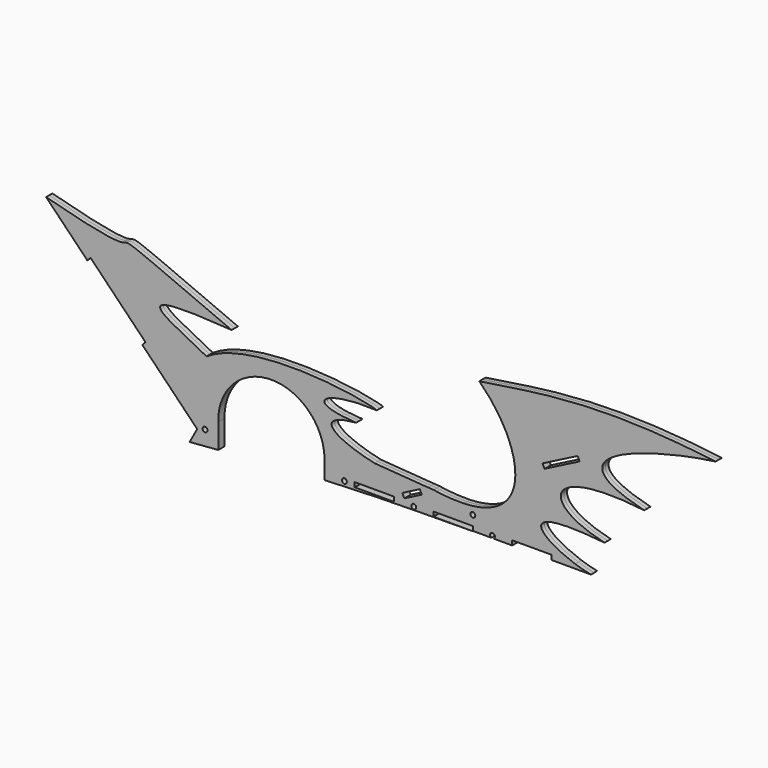
from build123d import *

# Parameters (mm, degrees)
F0_R     = 1.5875
F1_DEPTH = 2.54
F2_DEPTH = 2.54


# Not quite as in the source:
# - a feature names something its author has since deleted; it is built from what else it names


with BuildPart() as f1:
    # F0 (on Front) → F1 (new body)
    with BuildSketch(Plane.XZ):
        with BuildLine():
            Line((-117.7666419361, -55.4287118418), (-109.9768313618, -55.4287118418))
            Line((-109.9768313618, -55.4287118418), (-109.9768313618, -47.0136375922))
            ThreePointArc((-109.9768313618, -47.0136375922), (-106.8885192596, -31.8588641059), (-97.4549951083, -19.6027043016))
            add(Edge.make_bspline(
                [(-117.5484094073, -12.1659971935), (-110.6681944827, -14.9321483823), (-103.9782175093, -17.3987240026), (-97.4549951083, -19.6027043016)],
                knots=[85.5800903731, 85.5800903731, 85.5800903731, 85.5800903731, 105.0897215055, 105.0897215055, 105.0897215055, 105.0897215055], degree=3))
            add(Edge.make_bspline(
                [(-221.0534861924, 44.6501588425), (-181.5698408099, 17.8661525637), (-147.728857773, -0.032119976), (-117.5484094073, -12.1659971935)],
                knots=[0, 0, 0, 0, 85.5800903731, 85.5800903731, 85.5800903731, 85.5800903731], degree=3))
            Line((-221.0534861924, 44.6501588425), (-194.470886592, 17.3559213832))
            Line((-194.470886592, 17.3559213832), (-192.3419360702, 19.429364152))
            Line((-192.3419360702, 19.429364152), (-156.8984699364, -16.9629524605))
            Line((-156.8984699364, -16.9629524605), (-159.0274204582, -19.0363952293))
            Line((-159.0274204582, -19.0363952293), (-123.5839543244, -55.4287118418))
            Line((-123.5839543244, -55.4287118418), (-119.2412667127, -55.4287118418))
            ThreePointArc((-119.2412667127, -55.4287118418), (-119.3254386011, -52.6643963439), (-116.9164543244, -54.0228218418))
            ThreePointArc((-116.9164543244, -54.0228218418), (-117.1455288266, -54.8443061184), (-117.7666419361, -55.4287118418))
        make_face()
        with BuildLine():
            ThreePointArc((-97.4549951083, -19.6027043016), (-67.2988267393, -12.8616988757), (-43.9640451784, -33.1181451176))
            add(Edge.make_bspline(
                [(-43.9640451784, -33.1181451176), (-32.0425687929, -35.1610667408), (-20.543079457, -36.5394679062), (-9.2562094033, -37.5830486955)],
                knots=[162.0898574654, 162.0898574654, 162.0898574654, 162.0898574654, 202.5442303334, 202.5442303334, 202.5442303334, 202.5442303334], degree=3))
            add(Edge.make_bspline(
                [(-21.0130102932, -18.435029313), (-47.6523786783, -20.7854453474), (-38.7050335474, -30.7782148652), (-9.2562094033, -37.5830486955)],
                knots=[0, 0, 0, 0, 22.4692904525, 22.4692904525, 22.4692904525, 22.4692904525], degree=3))
            add(Edge.make_bspline(
                [(-7.7310134657, -7.0962994359), (-41.7368360795, -5.3299111314), (-56.8069815636, -16.3296777755), (-21.0130102932, -18.435029313)],
                knots=[0, 0, 0, 0, 17.4636260539, 17.4636260539, 17.4636260539, 17.4636260539], degree=3))
            add(Edge.make_bspline(
                [(-117.5484094073, -12.1659971935), (-86.6610095747, 8.189654137), (-15.093958471, -3.4407672938), (-7.7310134657, -7.0962994359)],
                knots=[0, 0, 0, 0, 109.9343544428, 109.9343544428, 109.9343544428, 109.9343544428], degree=3))
            add(Edge.make_bspline(
                [(-117.5484094073, -12.1659971935), (-110.6681944827, -14.9321483823), (-103.9782175093, -17.3987240026), (-97.4549951083, -19.6027043016)],
                knots=[85.5800903731, 85.5800903731, 85.5800903731, 85.5800903731, 105.0897215055, 105.0897215055, 105.0897215055, 105.0897215055], degree=3))
        make_face()
        with BuildLine():
            Line((-27.9141419361, -55.4287118418), (-21.9839543244, -55.4287118418))
            Line((-21.9839543244, -55.4287118418), (-21.9839543244, -52.4569118418))
            Line((-21.9839543244, -52.4569118418), (3.4160456756, -52.4569118418))
            Line((3.4160456756, -52.4569118418), (3.4160456756, -55.4287118418))
            Line((3.4160456756, -55.4287118418), (15.3787332873, -55.4287118418))
            ThreePointArc((15.3787332873, -55.4287118418), (15.2945613989, -52.6643963439), (17.7035456756, -54.0228218418))
            ThreePointArc((17.7035456756, -54.0228218418), (17.4744711734, -54.8443061184), (16.8533580639, -55.4287118418))
            Line((16.8533580639, -55.4287118418), (28.8160456756, -55.4287118418))
            Line((28.8160456756, -55.4287118418), (28.8160456756, -52.6365224585))
            Line((28.8160456756, -52.6365224585), (54.2160456756, -52.6365224585))
            Line((54.2160456756, -52.6365224585), (54.2160456756, -55.4287118418))
            Line((54.2160456756, -55.4287118418), (66.1787332873, -55.4287118418))
            ThreePointArc((66.1787332873, -55.4287118418), (66.0945613989, -52.6643963439), (68.5035456756, -54.0228218418))
            ThreePointArc((68.5035456756, -54.0228218418), (68.2744711734, -54.8443061184), (67.6533580639, -55.4287118418))
            Line((67.6533580639, -55.4287118418), (79.6160456756, -55.4287118418))
            Line((79.6160456756, -55.4287118418), (79.6160456756, -52.4715288512))
            Line((79.6160456756, -52.4715288512), (105.0160456756, -52.4715288512))
            Line((105.0160456756, -52.4715288512), (105.0160456756, -55.4287118418))
            Line((105.0160456756, -55.4287118418), (130.4160456756, -55.4287118418))
            add(Edge.make_bspline(
                [(130.4160456756, -55.4287118418), (127.0833152181, -54.7907548199), (123.567769086, -53.8343331493), (120.1337166001, -52.6704820922)],
                knots=[0, 0, 0, 0, 2.981631712, 2.981631712, 2.981631712, 2.981631712], degree=3))
            add(Edge.make_bspline(
                [(48.3758309171, -41.6905821706), (71.0941321723, -43.4592939375), (94.4273288023, -46.1963068791), (120.1337166001, -52.6704820922)],
                knots=[272.3833290429, 272.3833290429, 272.3833290429, 272.3833290429, 354.6125504281, 354.6125504281, 354.6125504281, 354.6125504281], degree=3))
            add(Edge.make_bspline(
                [(48.3758309171, -41.6905821706), (43.2278307913, -41.8740335792), (37.4162620901, -41.5445708983), (30.8966081292, -40.6238344152)],
                knots=[68.7701344649, 68.7701344649, 68.7701344649, 68.7701344649, 76.3944524282, 76.3944524282, 76.3944524282, 76.3944524282], degree=3))
            Line((30.8966081292, -40.6238344152), (21.3371492148, -45.5034172427))
            Line((21.3371492148, -45.5034172427), (10.0255792014, -51.277357304))
            Line((10.0255792014, -51.277357304), (8.674477227, -48.6304499209))
            Line((8.674477227, -48.6304499209), (19.9860472404, -42.8565098596))
            Line((19.9860472404, -42.8565098596), (25.3584616646, -40.1141850689))
            add(Edge.make_bspline(
                [(-9.2562094033, -37.5830486955), (2.4325313973, -38.6637863394), (13.8932426879, -39.3854364842), (25.3584616646, -40.1141850689)],
                knots=[202.5442303334, 202.5442303334, 202.5442303334, 202.5442303334, 244.4389873788, 244.4389873788, 244.4389873788, 244.4389873788], degree=3))
            add(Edge.make_bspline(
                [(-43.9640451784, -33.1181451176), (-32.0425687929, -35.1610667408), (-20.543079457, -36.5394679062), (-9.2562094033, -37.5830486955)],
                knots=[162.0898574654, 162.0898574654, 162.0898574654, 162.0898574654, 202.5442303334, 202.5442303334, 202.5442303334, 202.5442303334], degree=3))
            ThreePointArc((-43.9640451784, -33.1181451176), (-42.0894588544, -39.308762747), (-41.4107711408, -45.7412741932))
            ThreePointArc((-41.4107711408, -45.7412741932), (-41.4093090413, -45.924090419), (-41.4088216702, -46.1069118418))
            ThreePointArc((-41.4088216702, -46.1069118418), (-41.4093090413, -46.2897332645), (-41.4107711408, -46.4725494903))
            Line((-41.4107711408, -46.4725494903), (-41.4107711408, -55.4287118418))
            Line((-41.4107711408, -55.4287118418), (-29.3887667127, -55.4287118418))
            ThreePointArc((-29.3887667127, -55.4287118418), (-29.4729386011, -52.6643963439), (-27.0639543244, -54.0228218418))
            ThreePointArc((-27.0639543244, -54.0228218418), (-27.2930288266, -54.8443061184), (-27.9141419361, -55.4287118418))
        make_face()
        with Locations((54.2160456756, -46.2865224585)):
            Circle(F0_R, mode=Mode.SUBTRACT)
        with BuildLine():
            Line((-109.9768313618, -62.8472353007), (-109.9768313618, -55.4287118418))
            Line((-109.9768313618, -55.4287118418), (-117.7666419361, -55.4287118418))
            ThreePointArc((-117.7666419361, -55.4287118418), (-118.5039543244, -55.6103218418), (-119.2412667127, -55.4287118418))
            Line((-119.2412667127, -55.4287118418), (-123.5839543244, -55.4287118418))
            Line((-123.5839543244, -55.4287118418), (-128.4894852792, -64.325979178))
            add(Edge.make_bspline(
                [(-128.4894852792, -64.325979178), (-121.7990702135, -63.8053858531), (-115.6687309059, -63.3129022925), (-109.9768313618, -62.8472353007)],
                knots=[0, 0, 0, 0, 19.3690037374, 19.3690037374, 19.3690037374, 19.3690037374], degree=3))
        make_face()
        with BuildLine():
            add(Edge.make_bspline(
                [(58.3871234256, 30.9589318931), (71.6334399841, 18.2907250781), (80.3919593775, 2.3020275424), (81.5074353868, -11.4531938545)],
                knots=[0, 0, 0, 0, 31.5527935417, 31.5527935417, 31.5527935417, 31.5527935417], degree=3))
            Line((81.5074353868, -11.4531938545), (99.1670373344, -2.4389294304))
            Line((99.1670373344, -2.4389294304), (121.7901773612, 9.1089506922))
            Line((121.7901773612, 9.1089506922), (123.1412793355, 6.4620433091))
            Line((123.1412793355, 6.4620433091), (100.5181393087, -5.0858368135))
            Line((100.5181393087, -5.0858368135), (81.6265885359, -14.7289439771))
            add(Edge.make_bspline(
                [(81.6265885359, -14.7289439771), (81.4775915143, -29.4114492672), (71.7901506946, -40.8562018599), (48.3758309171, -41.6905821706)],
                knots=[34.0929366176, 34.0929366176, 34.0929366176, 34.0929366176, 68.7701344649, 68.7701344649, 68.7701344649, 68.7701344649], degree=3))
            add(Edge.make_bspline(
                [(48.3758309171, -41.6905821706), (71.0941321723, -43.4592939375), (94.4273288023, -46.1963068791), (120.1337166001, -52.6704820922)],
                knots=[272.3833290429, 272.3833290429, 272.3833290429, 272.3833290429, 354.6125504281, 354.6125504281, 354.6125504281, 354.6125504281], degree=3))
            add(Edge.make_bspline(
                [(120.1337166001, -52.6704820922), (97.4196175935, -44.9723387909), (78.2708583399, -28.1991783341), (139.1727849841, -34.4821810722)],
                knots=[2.981631712, 2.981631712, 2.981631712, 2.981631712, 22.7032516305, 22.7032516305, 22.7032516305, 22.7032516305], degree=3))
            add(Edge.make_bspline(
                [(139.1727849841, -34.4821810722), (96.3281169534, -24.4673900306), (100.2230867743, 0), (164.7682860494, -7.7760731801)],
                knots=[0, 0, 0, 0, 36.9911593969, 36.9911593969, 36.9911593969, 36.9911593969], degree=3))
            add(Edge.make_bspline(
                [(164.7682860494, -7.7760731801), (99.6666625142, 8.3588659763), (166.8688207865, 28.8012474775), (210.8263075352, 34.9213965237)],
                knots=[0, 0, 0, 0, 62.8045799468, 62.8045799468, 62.8045799468, 62.8045799468], degree=3))
            add(Edge.make_bspline(
                [(58.3871234256, 30.9589318931), (96.6607186991, 36.5597531199), (134.1467499733, 44.6605086327), (210.8263075352, 34.9213965237)],
                knots=[0, 0, 0, 0, 152.4906750524, 152.4906750524, 152.4906750524, 152.4906750524], degree=3))
        make_face()
        with BuildLine():
            add(Edge.make_bspline(
                [(-221.0534861924, 44.6501588425), (-181.5698408099, 17.8661525637), (-147.728857773, -0.032119976), (-117.5484094073, -12.1659971935)],
                knots=[0, 0, 0, 0, 85.5800903731, 85.5800903731, 85.5800903731, 85.5800903731], degree=3))
            add(Edge.make_bspline(
                [(-101.3629883528, 8.0616753548), (-179.9046397209, 13.7252416462), (-139.0098333359, 0), (-117.5484094073, -12.1659971935)],
                knots=[0, 0, 0, 0, 25.9061110828, 25.9061110828, 25.9061110828, 25.9061110828], degree=3))
            add(Edge.make_bspline(
                [(-221.0534861924, 44.6501588425), (-123.9654645324, 18.4180028737), (-220.0758159161, 58.7708987296), (-101.3629883528, 8.0616753548)],
                knots=[0, 0, 0, 0, 125.1580296945, 125.1580296945, 125.1580296945, 125.1580296945], degree=3))
        make_face()
        with BuildLine():
            Line((3.4160456756, -55.4287118418), (-21.9839543244, -55.4287118418))
            Line((-21.9839543244, -55.4287118418), (-27.9141419361, -55.4287118418))
            ThreePointArc((-27.9141419361, -55.4287118418), (-28.6514543244, -55.6103218418), (-29.3887667127, -55.4287118418))
            Line((-29.3887667127, -55.4287118418), (-41.4107711408, -55.4287118418))
            Line((-41.4107711408, -55.4287118418), (-41.4107711408, -57.6664364359))
            add(Edge.make_bspline(
                [(-41.4107711408, -57.6664364359), (-19.3143753017, -56.518291513), (7.3247499194, -55.8879261312), (54.2160456756, -55.6083224585)],
                knots=[117.4965318046, 117.4965318046, 117.4965318046, 117.4965318046, 215.4019720603, 215.4019720603, 215.4019720603, 215.4019720603], degree=3))
            Line((54.2160456756, -55.6083224585), (28.8160456756, -55.6083224585))
            Line((28.8160456756, -55.6083224585), (28.8160456756, -55.4287118418))
            Line((28.8160456756, -55.4287118418), (16.8533580639, -55.4287118418))
            ThreePointArc((16.8533580639, -55.4287118418), (16.1160456756, -55.6103218418), (15.3787332873, -55.4287118418))
            Line((15.3787332873, -55.4287118418), (3.4160456756, -55.4287118418))
        make_face()
        with BuildLine():
            Line((99.1670373344, -2.4389294304), (81.5074353868, -11.4531938545))
            add(Edge.make_bspline(
                [(81.5074353868, -11.4531938545), (81.5972362679, -12.5605516021), (81.6375027324, -13.653434234), (81.6265885359, -14.7289439771)],
                knots=[31.5527935417, 31.5527935417, 31.5527935417, 31.5527935417, 34.0929366176, 34.0929366176, 34.0929366176, 34.0929366176], degree=3))
            Line((81.6265885359, -14.7289439771), (100.5181393087, -5.0858368135))
            Line((100.5181393087, -5.0858368135), (99.1670373344, -2.4389294304))
        make_face()
        with BuildLine():
            add(Edge.make_bspline(
                [(25.3584616646, -40.1141850689), (26.5865600609, -40.1922450667), (27.8147101768, -40.2703865095), (29.0431978008, -40.3490594404)],
                knots=[244.4389873788, 244.4389873788, 244.4389873788, 244.4389873788, 248.926549635, 248.926549635, 248.926549635, 248.926549635], degree=3))
            Line((25.3584616646, -40.1141850689), (19.9860472404, -42.8565098596))
            Line((19.9860472404, -42.8565098596), (21.3371492148, -45.5034172427))
            Line((21.3371492148, -45.5034172427), (30.8966081292, -40.6238344152))
            add(Edge.make_bspline(
                [(30.8966081292, -40.6238344152), (30.2850473312, -40.537466896), (29.6672561358, -40.4458967962), (29.0431978008, -40.3490594404)],
                knots=[76.3944524282, 76.3944524282, 76.3944524282, 76.3944524282, 77.1096336335, 77.1096336335, 77.1096336335, 77.1096336335], degree=3))
        make_face()
    extrude(amount=F1_DEPTH)

    # F2 (add): faces of the model
    f2_faces = [f1.faces().sort_by_distance(p)[0] for p in [
        (-154.855246678, -2.54, -21.1905679866),
        (-154.855246678, 0, -21.1905679866),
    ]]
    extrude(f2_faces, amount=F2_DEPTH, dir=(0, -1, 0))


solid = f1.part
